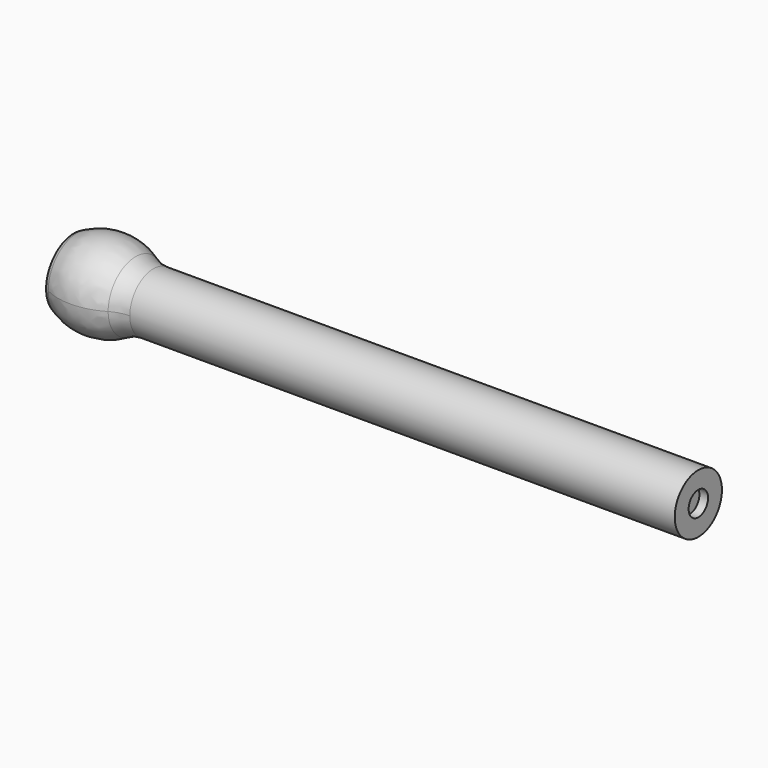
from build123d import *

# Parameters (mm, degrees)
F0_R      = 4.318
F1_DEPTH  = 81.28
F2_R      = 1.778
F3_DEPTH  = 1.27
F5_R      = 7.62
F6_FACE_R = 7.62
F8_R      = 5.08
F10_R     = 8.89
F11_R     = 5.08


with BuildPart() as f1:
    # F0 (on Right) → F1 (new body)
    with BuildSketch(Plane.YZ):
        Circle(F0_R)
    extrude(amount=F1_DEPTH)

    # F2 (on face) → F3 (cut)
    with BuildSketch(Plane.YZ.offset(81.28)):
        Circle(F2_R)
    extrude(amount=-F3_DEPTH, mode=Mode.SUBTRACT)

    # F0 (on Right) → F6 section 0
    with BuildSketch(Plane.YZ):
        Circle(F0_R)
    # F5 (on offset) → F6 section 1
    with BuildSketch(Plane.YZ.offset(-5.08)):
        Circle(F5_R)
    loft()

    # F6_face (on face) → F9 section 0
    with BuildSketch(Plane(origin=(-5.08, 0, 0), x_dir=(0, -1, 0), z_dir=(-1, 0, 0))):
        Circle(F6_FACE_R)
    # F8 (on offset) → F9 section 1
    with BuildSketch(Plane.YZ.offset(-10.16)):
        Circle(F8_R)
    loft()

    # F10
    f10_edges = [f1.edges().sort_by_distance(p)[0] for p in [
        (-5.08, 0, 7.62),
        (-5.08, 0, -7.62),
    ]]
    fillet(f10_edges, radius=F10_R)

    # F11
    f11_edges = [f1.edges().sort_by_distance(p)[0] for p in [
        (0, -4.318, 0),
    ]]
    fillet(f11_edges, radius=F11_R)


solid = f1.part
